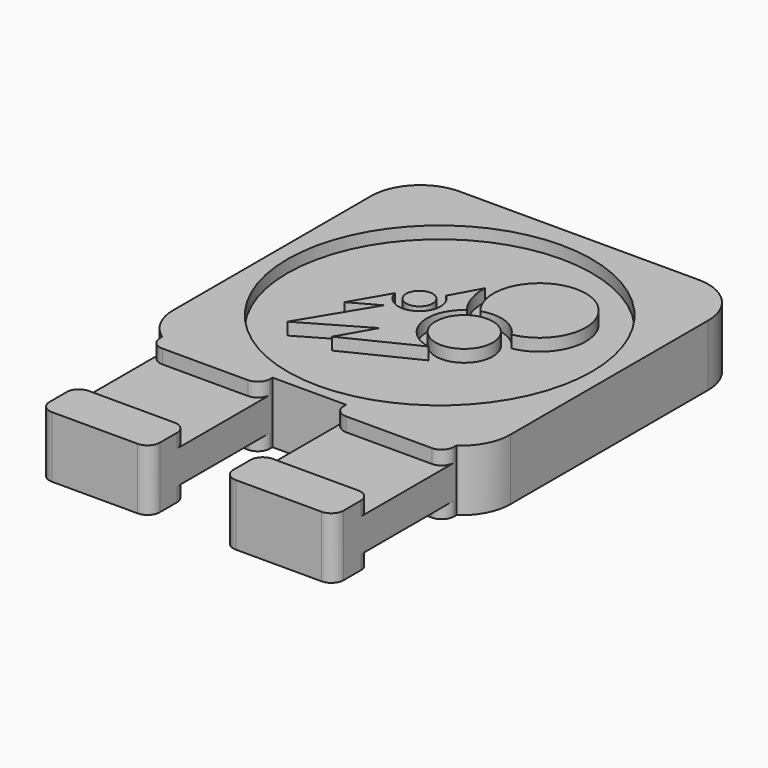
from build123d import *

# Parameters (mm, degrees)
F1_DEPTH    = 3.175
F2_W        = 9.525
F2_H        = 1.4478
F3_DEPTH    = 25.4
F4_R        = 15.7740752149
F4_R_2      = 2.9681243023
F4_R_3      = 1.3729847112
F5_DEPTH    = 1.27
F6_T1_DEPTH = 31.75
F6_T3_DEPTH = 27.3506510316
F7_R        = 1.27


# Not quite as in the source:
# - a fillet or chamfer that OpenCascade refuses, or shapes differently, is made with other operations: its cross-section is extruded or revolved along the edge and cut away or added


with BuildPart() as f1:
    # F0 (on Top) → F1 (new body, symmetric)
    with BuildSketch(Plane.XY):
        Polygon((17.7787664203, 21.9838270611), (-17.1462335797, 21.9838270611), (-17.1462335797, -12.9411729389), (-14.9237335797, -12.9411729389), (-14.9237335797, -28.8161729389), (-3.4937335797, -28.8161729389), (-3.4937335797, -12.9411729389), (4.1262664203, -12.9411729389), (4.1262664203, -28.8161729389), (15.5562664203, -28.8161729389), (15.5562664203, -12.9411729389), (17.7787664203, -12.9411729389), align=None)
    extrude(amount=F1_DEPTH, both=True)

    # F2 (on Right) → F3 (cut, symmetric)
    with BuildSketch(Plane.YZ):
        with Locations((-19.2911729389, -2.4511)):
            Rectangle(F2_W, F2_H)
        with Locations((-19.2911729389, 2.4511)):
            Rectangle(F2_W, F2_H)
    extrude(amount=F3_DEPTH, both=True, mode=Mode.SUBTRACT)

    # F4 (on face) → F5 (cut)
    with BuildSketch(Plane.XY.offset(3.175)):
        with Locations((0.2568493655, 4.0185162798)):
            Circle(F4_R)
        with BuildLine():
            Line((-1.5064536128, 7.0266816765), (0.1482767001, 10.0501550651))
            ThreePointArc((0.1482767001, 10.0501550651), (0.4096706183, 7.9792062399), (1.3765677405, 6.1292695458))
            ThreePointArc((1.3765677405, 6.1292695458), (-0.1382695754, 2.1387635418), (2.9542085605, -0.8032509449))
            Line((2.9542085605, -0.8032509449), (-4.2190060268, -4.3320505521))
            Line((-4.2190060268, -4.3320505521), (-2.1576185001, -0.7580867248))
            Line((-2.1576185001, -0.7580867248), (-8.6794582017, -4.5345938661))
            Line((-8.6794582017, -4.5345938661), (-4.3788731984, 2.5767316464))
            Line((-4.3788731984, 2.5767316464), (-7.1943101482, 1.0284683409))
            Line((-7.1943101482, 1.0284683409), (-4.9999261676, 4.815935468))
            ThreePointArc((-4.9999261676, 4.815935468), (-1.6824509255, 3.4391903431), (-1.5064536128, 7.0266816765))
        make_face(mode=Mode.SUBTRACT)
        with Locations((3.6213599069, 2.9943462909)):
            Circle(F4_R_2, mode=Mode.SUBTRACT)
        with Locations((-2.8567614499, 5.2948631346)):
            Circle(F4_R_3, mode=Mode.SUBTRACT)
        with BuildLine():
            ThreePointArc((2.3814487819, 6.6452990552), (7.6456545146, 14.2492672348), (6.8950720548, 5.0314139032))
            ThreePointArc((6.8950720548, 5.0314139032), (4.9195289911, 6.6249926126), (2.3814487819, 6.6452990552))
        make_face(mode=Mode.SUBTRACT)
    extrude(amount=-F5_DEPTH, mode=Mode.SUBTRACT)

    # F6: fillet of radius 5.08 on 4 edges, made by hand

    # F6_s2 → F6_t1 (cut)
    with BuildSketch(Plane.XY.offset(-15.875)):
        with BuildLine():
            ThreePointArc((12.6987664203, 21.9838270611), (16.2908688687, 20.4959295096), (17.7787664203, 16.9038270611))
            Line((17.7787664203, 16.9038270611), (17.7787664203, 21.9838270611))
            Line((17.7787664203, 21.9838270611), (12.6987664203, 21.9838270611))
        make_face()
        with BuildLine():
            ThreePointArc((-17.1462335797, 16.9038270611), (-15.6583360282, 20.4959295096), (-12.0662335797, 21.9838270611))
            Line((-12.0662335797, 21.9838270611), (-17.1462335797, 21.9838270611))
            Line((-17.1462335797, 21.9838270611), (-17.1462335797, 16.9038270611))
        make_face()
    extrude(amount=F6_T1_DEPTH, mode=Mode.SUBTRACT)

    # F6_s4 → F6_t3 (cut)
    with BuildSketch(Plane.XY.offset(-13.6753255158)):
        with BuildLine():
            ThreePointArc((-14.9237335797, -12.9411729388), (-16.5563616403, -11.1169951731), (-17.1462335797, -8.7410427325))
            Line((-17.1462335797, -8.7410427325), (-17.1462335797, -12.9411729389))
            Line((-17.1462335797, -12.9411729389), (-14.9237335797, -12.9411729388))
        make_face()
        with BuildLine():
            ThreePointArc((17.7787664203, -8.7410427325), (17.1888944808, -11.1169951731), (15.5562664203, -12.9411729388))
            Line((15.5562664203, -12.9411729388), (17.7787664203, -12.9411729389))
            Line((17.7787664203, -12.9411729389), (17.7787664203, -8.7410427325))
        make_face()
    extrude(amount=F6_T3_DEPTH, mode=Mode.SUBTRACT)

    # F7
    f7_edges = [f1.edges().sort_by_distance(p)[0] for p in [
        (-14.923734, -14.528673, 2.4511),
        (-3.493734, -14.528673, 2.4511),
        (15.556266, -14.528673, 2.4511),
        (4.126266, -14.528673, 2.4511),
        (15.556266, -14.528673, -2.4511),
        (4.126266, -14.528673, -2.4511),
        (-14.923734, -14.528673, -2.4511),
        (-3.493734, -14.528673, -2.4511),
        (-3.493734, -24.053673, -2.4511),
        (-3.493734, -24.053673, 2.4511),
        (15.556266, -24.053673, -2.4511),
        (15.556266, -24.053673, 2.4511),
        (15.556266, -28.816173, 0),
        (4.126266, -28.816173, 0),
        (-3.493734, -28.816173, 0),
        (-14.923734, -28.816173, 0),
        (-14.923734, -24.053673, 2.4511),
        (-14.923734, -24.053673, -2.4511),
        (4.126266, -24.053673, 2.4511),
        (4.126266, -24.053673, -2.4511),
    ]]
    fillet(f7_edges, radius=F7_R)


solid = f1.part
